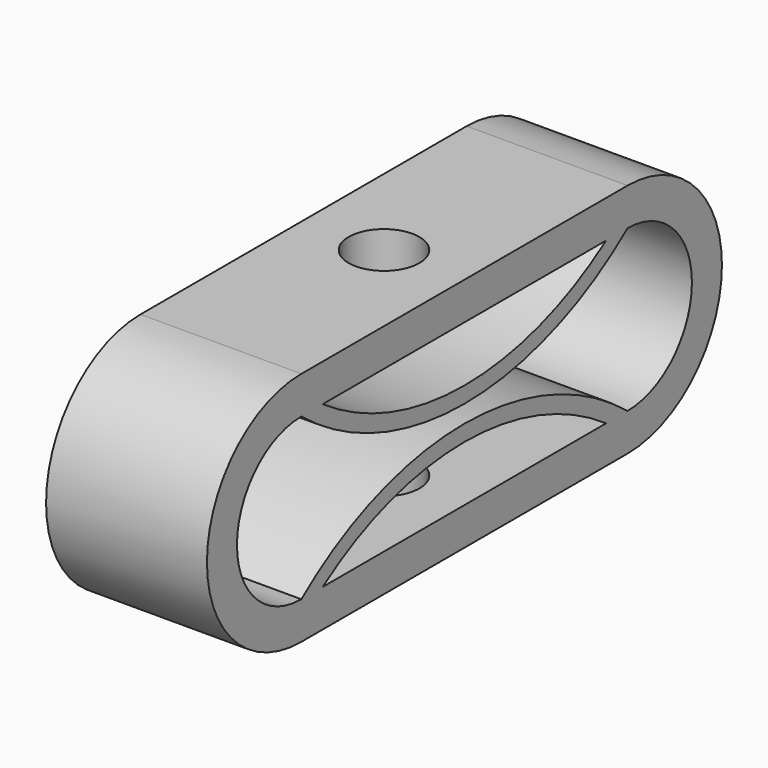
from build123d import *

# Parameters (mm, degrees)
F1_DEPTH = 7.5
F3_D     = 6.6
F3_DEPTH = 4
F3_TIP   = 1.9828400428


# Not quite as in the source:
# - a pattern or mirror of a feature is missing from the dataset's text; its kind, count and spacing are read off the source's solid


with BuildPart() as f1:
    # F0 (on Right) → F1 (new body, symmetric)
    with BuildSketch(Plane.YZ):
        with BuildLine():
            Line((19.0101097905, 11), (-19.0101097905, 11))
            ThreePointArc((-19.0101097905, 11), (-30.0101097905, 0), (-19.0101097905, -11))
            Line((-19.0101097905, -11), (19.0101097905, -11))
            ThreePointArc((19.0101097905, -11), (30.0101097905, 0), (19.0101097905, 11))
        make_face()
        with BuildLine():
            Line((16.508441914, -7.5), (-16.508441914, -7.5))
            ThreePointArc((-16.508441914, -7.5), (0, -2.3140263028), (16.508441914, -7.5))
        make_face(mode=Mode.SUBTRACT)
        with BuildLine():
            ThreePointArc((-19.0101097905, -7.5), (-26.5101097905, 0), (-19.0101097905, 7.5))
            ThreePointArc((-19.0101097905, 7.5), (0, 0.8140263028), (19.0101097905, 7.5))
            ThreePointArc((19.0101097905, 7.5), (26.5101097905, 0), (19.0101097905, -7.5))
            ThreePointArc((19.0101097905, -7.5), (0, -0.8140263028), (-19.0101097905, -7.5))
        make_face(mode=Mode.SUBTRACT)
        with BuildLine():
            ThreePointArc((16.508441914, 7.5), (0, 2.3140263028), (-16.508441914, 7.5))
            Line((-16.508441914, 7.5), (16.508441914, 7.5))
        make_face(mode=Mode.SUBTRACT)
    extrude(amount=F1_DEPTH, both=True)

    # F3
    with Locations(Plane.XY.offset(11)):
        with Locations((0, 0)):
            f3 = Hole(F3_D / 2, depth=F3_DEPTH)
            with Locations((0, 0, -(F3_DEPTH + F3_TIP / 2))):  # 118° drill point
                Cone(0, F3_D / 2, F3_TIP, mode=Mode.SUBTRACT)

    # F3_copies: F3 across plane
    add(f3.mirror(Plane(origin=(0, 0, 0), x_dir=(-1, 0, 0), z_dir=(0, 0, -1))), mode=Mode.SUBTRACT)


solid = f1.part
